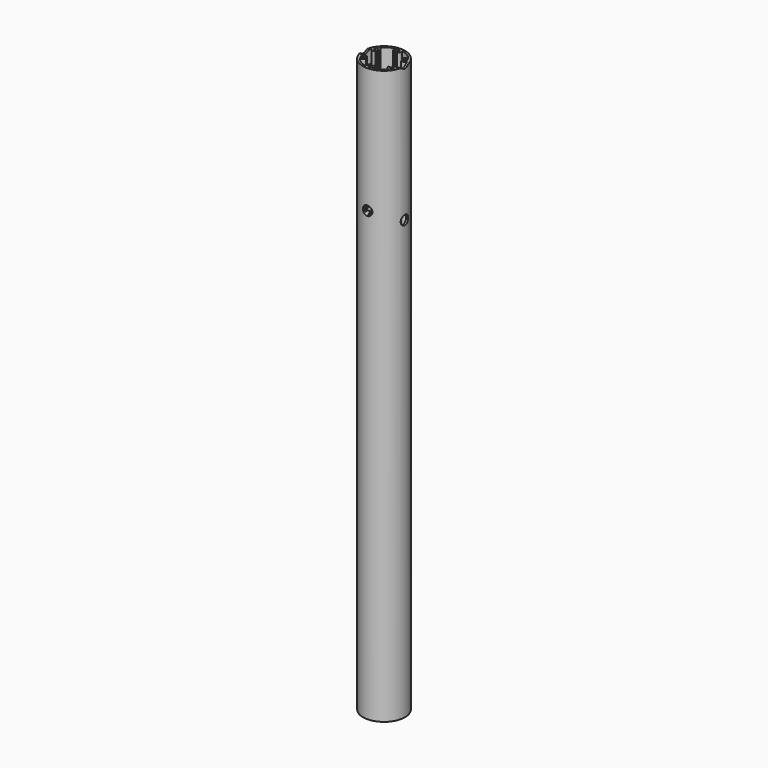
from build123d import *

# Parameters (mm, degrees)
F0_R           = 31.75
F0_R_2         = 28.75
F1_DEPTH       = 868
F2_R           = 5.5
F2_R_2         = 2.5
F3_DEPTH       = 868
F5_DEPTH       = 868.001
F7_DEPTH       = 31.751
F7_DEPTH_BACK  = 31.751
F8_T4_DEPTH    = 17.4404652914
F8_S5_R        = 5.5
F8_T6_DEPTH    = 11
F8_T10_DEPTH   = 17.4404652914
F8_S11_R       = 28.75
F8_T12_DEPTH   = 11
F8_T16_DEPTH   = 17.4404652914
F8_S17_R       = 28.75
F8_T18_DEPTH   = 11
F8_T22_DEPTH   = 17.4404652914
F8_S23_R       = 5.5
F8_T24_DEPTH   = 11
F9_R           = 7.15
F10_DEPTH      = 31.7510001
F10_DEPTH_BACK = 31.7510001
F11_R          = 7.15
F12_DEPTH      = 31.7510001
F12_DEPTH_BACK = 31.7510001


# Not quite as in the source:
# - a fillet or chamfer that OpenCascade refuses, or shapes differently, is made with other operations: its cross-section is extruded or revolved along the edge and cut away or added


with BuildPart() as f1:
    # F0 (on Top) → F1 (new body)
    with BuildSketch(Plane.XY):
        Circle(F0_R)
        Circle(F0_R_2, mode=Mode.SUBTRACT)
    extrude(amount=F1_DEPTH)

    # F2 (on Top) → F3 (join, through all)
    with BuildSketch(Plane.XY):
        with Locations((0, 25.75)):
            Circle(F2_R)
        with Locations((0, 25.75)):
            Circle(F2_R_2, mode=Mode.SUBTRACT)
        with Locations((-22.3001541474, 12.875)):
            Circle(F2_R)
        with Locations((-22.3001541474, 12.875)):
            Circle(F2_R_2, mode=Mode.SUBTRACT)
        with Locations((-22.3001541474, -12.875)):
            Circle(F2_R)
        with Locations((-22.3001541474, -12.875)):
            Circle(F2_R_2, mode=Mode.SUBTRACT)
        with Locations((0, -25.75)):
            Circle(F2_R)
        with Locations((0, -25.75)):
            Circle(F2_R_2, mode=Mode.SUBTRACT)
        with Locations((22.3001541474, -12.875)):
            Circle(F2_R)
        with Locations((22.3001541474, -12.875)):
            Circle(F2_R_2, mode=Mode.SUBTRACT)
        with Locations((22.3001541474, 12.875)):
            Circle(F2_R)
        with Locations((22.3001541474, 12.875)):
            Circle(F2_R_2, mode=Mode.SUBTRACT)
    extrude(amount=F3_DEPTH)

    # F4 (on Top) → F5 (cut, through all)
    with BuildSketch(Plane.XY):
        with BuildLine():
            Line((0, 25.75), (-2.75, 20.9868602792))
            ThreePointArc((-2.75, 20.9868602792), (0, 20.25), (2.75, 20.9868602792))
            Line((2.75, 20.9868602792), (0, 25.75))
        make_face()
        with BuildLine():
            Line((-16.8001541474, 12.875), (-22.3001541474, 12.875))
            Line((-22.3001541474, 12.875), (-19.5501541474, 8.1118602792))
            ThreePointArc((-19.5501541474, 8.1118602792), (-17.5370144266, 10.125), (-16.8001541474, 12.875))
        make_face()
        with BuildLine():
            Line((-19.5501541474, -8.1118602792), (-22.3001541474, -12.875))
            Line((-22.3001541474, -12.875), (-16.8001541474, -12.875))
            ThreePointArc((-16.8001541474, -12.875), (-17.5370144266, -10.125), (-19.5501541474, -8.1118602792))
        make_face()
        with BuildLine():
            Line((-2.75, -20.9868602792), (0, -25.75))
            Line((0, -25.75), (2.75, -20.9868602792))
            ThreePointArc((2.75, -20.9868602792), (0, -20.25), (-2.75, -20.9868602792))
        make_face()
        with BuildLine():
            Line((16.8001541474, -12.875), (22.3001541474, -12.875))
            Line((22.3001541474, -12.875), (19.5501541474, -8.1118602792))
            ThreePointArc((19.5501541474, -8.1118602792), (17.5370144266, -10.125), (16.8001541474, -12.875))
        make_face()
        with BuildLine():
            Line((19.5501541474, 8.1118602792), (22.3001541474, 12.875))
            Line((22.3001541474, 12.875), (16.8001541474, 12.875))
            ThreePointArc((16.8001541474, 12.875), (17.5370144266, 10.125), (19.5501541474, 8.1118602792))
        make_face()
    extrude(amount=F5_DEPTH, mode=Mode.SUBTRACT)

    # F6 (on Right) → F7 (cut, two sides)
    with BuildSketch(Plane.YZ) as f7_sk:
        with BuildLine():
            Line((5.862387447, 868), (-5.862387447, 868))
            ThreePointArc((-5.862387447, 868), (0, 864.5), (5.862387447, 868))
        make_face()
    extrude(amount=-F7_DEPTH, mode=Mode.SUBTRACT)
    extrude(f7_sk.sketch, amount=F7_DEPTH_BACK, mode=Mode.SUBTRACT)

    # F8: fillet of radius 6 on 4 edges, made by hand


with BuildPart() as f8_tool2:
    # F8_s3 → F8_t4 (new body)
    with BuildSketch(Plane.YZ.offset(-20.9547884557)):
        with BuildLine():
            ThreePointArc((-4.5971047614, 866.3411870524), (-6.508061671, 867.5698798153), (-8.7388549924, 868))
            Line((-8.7388549924, 868), (-5.862387447, 868))
            ThreePointArc((-5.862387447, 868), (-5.2951071201, 867.1207385008), (-4.5971047614, 866.3411870524))
        make_face()
    extrude(amount=-F8_T4_DEPTH)

    # F8_s5 → F8_t6 (cut, symmetric)
    with BuildSketch(Plane.XY.offset(867.2)):
        with Locations((-22.3001541474, -12.875)):
            Circle(F8_S5_R)
    extrude(amount=F8_T6_DEPTH, both=True, mode=Mode.SUBTRACT)


with BuildPart() as f1_1:
    add(f1.part)

    # F8_t1: cut F8_tool2
    add(f8_tool2.part, mode=Mode.SUBTRACT)


with BuildPart() as f8_tool8:
    # F8_s9 → F8_t10 (new body)
    with BuildSketch(Plane.YZ.offset(38.3952537472)):
        with BuildLine():
            ThreePointArc((-8.7388549924, 868), (-6.508061671, 867.5698798153), (-4.5971047614, 866.3411870524))
            ThreePointArc((-4.5971047614, 866.3411870524), (-5.2951071201, 867.1207385008), (-5.862387447, 868))
            Line((-5.862387447, 868), (-8.7388549924, 868))
        make_face()
    extrude(amount=-F8_T10_DEPTH)

    # F8_s11 → F8_t12 (cut, symmetric)
    with BuildSketch(Plane.XY.offset(867.2)):
        Circle(F8_S11_R)
    extrude(amount=F8_T12_DEPTH, both=True, mode=Mode.SUBTRACT)


with BuildPart() as f1_2:
    add(f1_1.part)

    # F8_t7: cut F8_tool8
    add(f8_tool8.part, mode=Mode.SUBTRACT)


with BuildPart() as f8_tool14:
    # F8_s15 → F8_t16 (new body)
    with BuildSketch(Plane.YZ.offset(20.9547884557)):
        with BuildLine():
            ThreePointArc((8.7388549924, 868), (6.508061671, 867.5698798153), (4.5971047614, 866.3411870524))
            ThreePointArc((4.5971047614, 866.3411870524), (5.2951071201, 867.1207385008), (5.862387447, 868))
            Line((5.862387447, 868), (8.7388549924, 868))
        make_face()
    extrude(amount=F8_T16_DEPTH)

    # F8_s17 → F8_t18 (cut, symmetric)
    with BuildSketch(Plane.XY.offset(867.2)):
        Circle(F8_S17_R)
    extrude(amount=F8_T18_DEPTH, both=True, mode=Mode.SUBTRACT)


with BuildPart() as f1_3:
    add(f1_2.part)

    # F8_t13: cut F8_tool14
    add(f8_tool14.part, mode=Mode.SUBTRACT)


with BuildPart() as f8_tool20:
    # F8_s21 → F8_t22 (new body)
    with BuildSketch(Plane.YZ.offset(-38.3952537472)):
        with BuildLine():
            ThreePointArc((8.7388549924, 868), (6.508061671, 867.5698798153), (4.5971047614, 866.3411870524))
            ThreePointArc((4.5971047614, 866.3411870524), (5.2951071201, 867.1207385008), (5.862387447, 868))
            Line((5.862387447, 868), (8.7388549924, 868))
        make_face()
    extrude(amount=F8_T22_DEPTH)

    # F8_s23 → F8_t24 (cut, symmetric)
    with BuildSketch(Plane.XY.offset(867.2)):
        with Locations((-22.3001541474, 12.875)):
            Circle(F8_S23_R)
    extrude(amount=F8_T24_DEPTH, both=True, mode=Mode.SUBTRACT)


with BuildPart() as f1_4:
    add(f1_3.part)

    # F8_t19: cut F8_tool20
    add(f8_tool20.part, mode=Mode.SUBTRACT)

    # F9 (on Right) → F10 (cut, two sides)
    with BuildSketch(Plane.YZ) as f10_sk:
        with Locations((0, 663)):
            Circle(F9_R)
    extrude(amount=-F10_DEPTH, mode=Mode.SUBTRACT)
    extrude(f10_sk.sketch, amount=F10_DEPTH_BACK, mode=Mode.SUBTRACT)

    # F11 (on Front) → F12 (cut, two sides)
    with BuildSketch(Plane.XZ) as f12_sk:
        with Locations((0, 678)):
            Circle(F11_R)
    extrude(amount=-F12_DEPTH, mode=Mode.SUBTRACT)
    extrude(f12_sk.sketch, amount=F12_DEPTH_BACK, mode=Mode.SUBTRACT)


solid = f1_4.part
